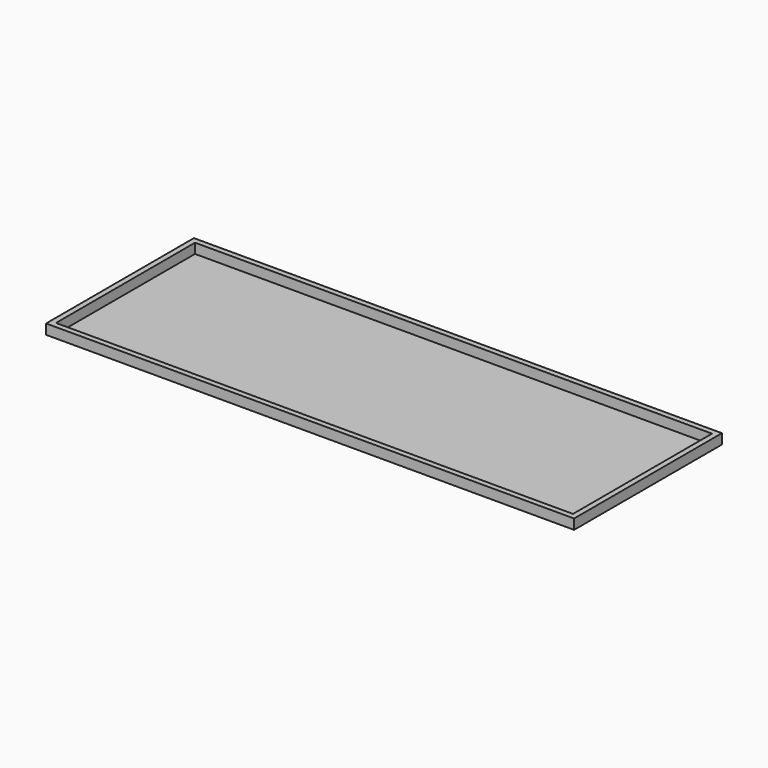
from build123d import *

# Parameters (mm, degrees)
F0_W     = 6096
F0_H     = 2133.6
F1_DEPTH = 1.5875
F2_W     = 63.5
F2_H     = 63.5
F2_W_2   = 5969
F2_H_2   = 2006.6
F3_DEPTH = 114.3


# Not quite as in the source:
# - a length typed as a fraction of an inch, garbled in the dataset ("3 / 203.2 mm" for 3/8 in), is restored


with BuildPart() as f1:
    # F0 (on Top) → F1 (new body)
    with BuildSketch(Plane.XY):
        with Locations((2064.3697643517, 48.2263118029)):
            Rectangle(F0_W, F0_H)
    extrude(amount=F1_DEPTH)

    # F2 (on face) → F3 (join)
    with BuildSketch(Plane.XY.offset(1.5875)):
        with Locations((5080.6197643517, 1083.2763118029)):
            Rectangle(F2_W, F2_H)
        with Locations((2064.3697643517, 1083.2763118029)):
            Rectangle(F2_W_2, F2_H)
        with Locations((5080.6197643517, 48.2263118029)):
            Rectangle(F2_W, F2_H_2)
        with Locations((-951.8802356483, 1083.2763118029)):
            Rectangle(F2_W, F2_H)
        with Locations((5080.6197643517, -986.8236881971)):
            Rectangle(F2_W, F2_H)
        with Locations((-951.8802356483, 48.2263118029)):
            Rectangle(F2_W, F2_H_2)
        with Locations((2064.3697643517, -986.8236881971)):
            Rectangle(F2_W_2, F2_H)
        with Locations((-951.8802356483, -986.8236881971)):
            Rectangle(F2_W, F2_H)
    extrude(amount=F3_DEPTH)


solid = f1.part
